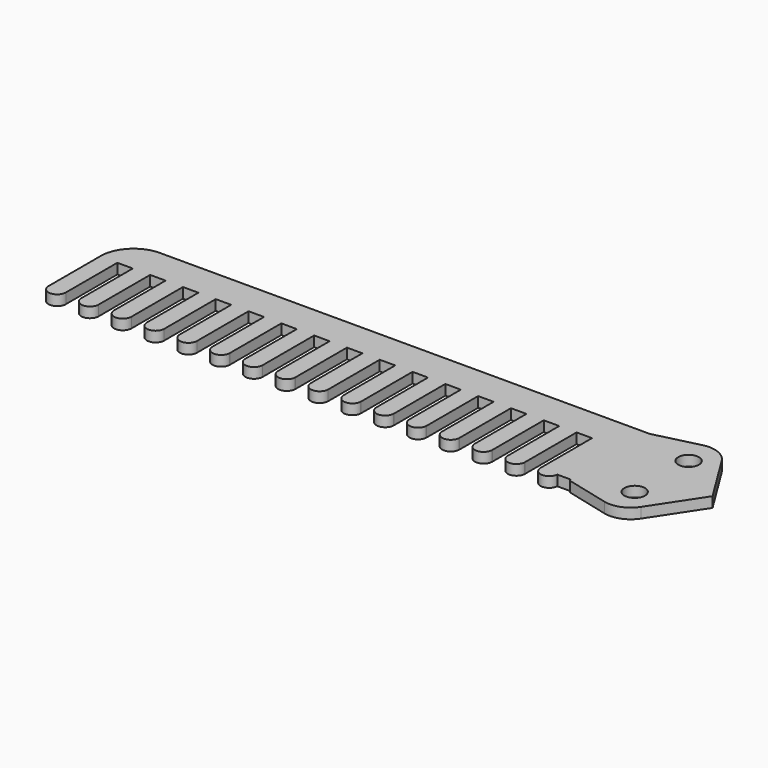
from build123d import *
from build123d import SkipClean  # not in build123d's __all__

# Parameters (mm, degrees)
F0_R     = 2
F1_DEPTH = 2
F3_DEPTH = 25.4
F4_DEPTH = 2
F5_DEPTH = 25.4


# Not quite as in the source:
# - a feature names something its author has since deleted; it is built from what else it names


with BuildPart() as f1:
    # F0 (on Top) → F1 (new body)
    with BuildSketch(Plane.XY):
        with BuildLine():
            ThreePointArc((-44.4982377637, 15.9537835574), (-46.6435438514, 15.0651686804), (-47.5321587284, 12.9198625927))
            Line((-47.5321587284, 12.9198625927), (-47.5321587284, 1.9581455603))
            ThreePointArc((-47.5321587284, 1.9581455603), (-46.0701489095, -1.5749303628), (-42.539108537, -3.0418496097))
            Line((-42.539108537, -3.0418496097), (58.6544047029, -3.182504855))
            ThreePointArc((58.6544047029, -3.182504855), (58.695576092, -3.383063352), (58.8128977225, -3.5508561677))
            Line((58.8128977225, -3.5508561677), (67.1425286707, -5.6492492557))
            ThreePointArc((67.1425286707, -5.6492492557), (70.1745553832, -5.4613941054), (72.5382215144, -3.553107449))
            Line((72.5382215144, -3.553107449), (78.7976136626, 5.9399087982))
            ThreePointArc((78.7976136626, 5.9399087982), (78.7234830832, 6.1327797263), (78.5951017421, 6.2946833056))
            Line((78.5951017421, 6.2946833056), (72.6648820615, 15.8458770867))
            ThreePointArc((72.6648820615, 15.8458770867), (70.3034587252, 17.8389512741), (67.2215312081, 18.0634232527))
            Line((67.2215312081, 18.0634232527), (58.6544042144, 15.9537835574))
            Line((58.6544042144, 15.9537835574), (-44.4982377637, 15.9537835574))
        make_face()
        with Locations((68.7303330245, -0.2896678891)):
            Circle(F0_R, mode=Mode.SUBTRACT)
        with Locations((68.7701961271, 12.7037232041)):
            Circle(F0_R, mode=Mode.SUBTRACT)
    extrude(amount=F1_DEPTH)

    # F2 (on face) → F3 (cut)
    with BuildSketch(Plane.XY.offset(2)):
        with BuildLine():
            Line((-10.789108537, 9.4149718061), (-13.784505137, 9.4149718061))
            Line((-13.784505137, 9.4149718061), (-13.784505137, -3.0465123845))
            ThreePointArc((-13.784505137, -3.0465123845), (-13.7845980378, -3.0641656349), (-13.7848767298, -3.0818169297))
            Line((-13.7848767298, -3.0818169297), (-10.7886505729, -3.0859815734))
            ThreePointArc((-10.7886505729, -3.0859815734), (-10.7890247148, -3.0639170979), (-10.789108537, -3.0418496097))
            Line((-10.789108537, -3.0418496097), (-10.789108537, 9.4149718061))
        make_face()
        with BuildLine():
            Line((-4.439108537, 9.4149718061), (-7.434505137, 9.4149718061))
            Line((-7.434505137, 9.4149718061), (-7.434505137, -3.0465123845))
            ThreePointArc((-7.434505137, -3.0465123845), (-7.4346503047, -3.0685795544), (-7.4350857828, -3.0906429046))
            Line((-7.4350857828, -3.0906429046), (-4.4384195675, -3.0948081599))
            ThreePointArc((-4.4384195675, -3.0948081599), (-4.4389730944, -3.0683316044), (-4.439108537, -3.0418496097))
            Line((-4.439108537, -3.0418496097), (-4.439108537, 9.4149718061))
        make_face()
        with BuildLine():
            Line((1.910891463, 9.4149718061), (-1.084505137, 9.4149718061))
            Line((-1.084505137, 9.4149718061), (-1.084505137, -3.0465123845))
            ThreePointArc((-1.084505137, -3.0465123845), (-1.0847141969, -3.0729939003), (-1.0853413245, -3.0994688148))
            Line((-1.0853413245, -3.0994688148), (1.911857947, -3.1036348111))
            ThreePointArc((1.911857947, -3.1036348111), (1.9110901561, -3.0727466615), (1.910891463, -3.0418496097))
            Line((1.910891463, -3.0418496097), (1.910891463, 9.4149718061))
        make_face()
        with BuildLine():
            Line((8.260891463, 9.4149718061), (5.265494863, 9.4149718061))
            Line((5.265494863, 9.4149718061), (5.265494863, -3.0465123845))
            ThreePointArc((5.265494863, -3.0465123845), (5.2652102793, -3.0774087645), (5.2643566248, -3.1082946604))
            Line((5.2643566248, -3.1082946604), (8.2622802241, -3.1124616635))
            ThreePointArc((8.2622802241, -3.1124616635), (8.2612141473, -3.0771629469), (8.260891463, -3.0418496097))
            Line((8.260891463, -3.0418496097), (8.260891463, 9.4149718061))
        make_face()
        with BuildLine():
            Line((14.610891463, 9.4149718061), (11.615494863, 9.4149718061))
            Line((11.615494863, 9.4149718061), (11.615494863, -3.0465123845))
            ThreePointArc((11.615494863, -3.0465123845), (11.6150740117, -3.0818246882), (11.6139098113, -3.1171203048))
            Line((11.6139098113, -3.1171203048), (14.6126631372, -3.1212884611))
            ThreePointArc((14.6126631372, -3.1212884611), (14.6113068287, -3.081579528), (14.610891463, -3.0418496097))
            Line((14.610891463, -3.0418496097), (14.610891463, 9.4149718061))
        make_face()
        with BuildLine():
            Line((17.9635023619, -3.1259460039), (20.9630926527, -3.1301153236))
            ThreePointArc((20.9630926527, -3.1301153236), (20.9614111694, -3.0859969529), (20.960891463, -3.0418496097))
            Line((20.960891463, -3.0418496097), (20.960891463, 9.4149718061))
            Line((20.960891463, 9.4149718061), (17.965494863, 9.4149718061))
            Line((17.965494863, 9.4149718061), (17.965494863, -3.0465123845))
            ThreePointArc((17.965494863, -3.0465123845), (17.9649690528, -3.0862409946), (17.9635023619, -3.1259460039))
        make_face()
        with BuildLine():
            Line((24.3130483101, -3.1347716382), (27.3135688072, -3.1389422508))
            ThreePointArc((27.3135688072, -3.1389422508), (27.3115271807, -3.0904153143), (27.310891463, -3.0418496097))
            Line((27.310891463, -3.0418496097), (27.310891463, 9.4149718061))
            Line((27.310891463, 9.4149718061), (24.315494863, 9.4149718061))
            Line((24.315494863, 9.4149718061), (24.315494863, -3.0465123845))
            ThreePointArc((24.315494863, -3.0465123845), (24.3148524325, -3.0906581124), (24.3130483101, -3.1347716382))
        make_face()
        with BuildLine():
            Line((30.6625476193, -3.1435972077), (33.6640916417, -3.147769243))
            ThreePointArc((33.6640916417, -3.147769243), (33.6616548753, -3.0948347051), (33.660891463, -3.0418496097))
            Line((33.660891463, -3.0418496097), (33.660891463, 9.4149718061))
            Line((33.660891463, 9.4149718061), (30.665494863, 9.4149718061))
            Line((30.665494863, 9.4149718061), (30.665494863, -3.0465123845))
            ThreePointArc((30.665494863, -3.0465123845), (30.6647241389, -3.0950761342), (30.6625476193, -3.1435972077))
        make_face()
        with BuildLine():
            Line((37.0120002484, -3.1524227123), (40.014661201, -3.1565963001))
            ThreePointArc((40.014661201, -3.1565963001), (40.011794267, -3.0992552184), (40.010891463, -3.0418496097))
            Line((40.010891463, -3.0418496097), (40.010891463, 9.4149718061))
            Line((40.010891463, 9.4149718061), (37.015494863, 9.4149718061))
            Line((37.015494863, 9.4149718061), (37.015494863, -3.0465123845))
            ThreePointArc((37.015494863, -3.0465123845), (37.0145841593, -3.0994951529), (37.0120002484, -3.1524227123))
        make_face()
        with BuildLine():
            Line((43.3614061528, -3.1612481519), (46.3652775338, -3.1654234222))
            ThreePointArc((46.3652775338, -3.1654234222), (46.361945371, -3.1036769476), (46.360891463, -3.0418496097))
            Line((46.360891463, -3.0418496097), (46.360891463, 9.4149718061))
            Line((46.360891463, 9.4149718061), (43.365494863, 9.4149718061))
            Line((43.365494863, 9.4149718061), (43.365494863, -3.0465123845))
            ThreePointArc((43.365494863, -3.0465123845), (43.3644324794, -3.1039152616), (43.3614061528, -3.1612481519))
        make_face()
        with BuildLine():
            Line((49.7107652838, -3.1700735266), (52.7159406928, -3.1742506094))
            ThreePointArc((52.7159406928, -3.1742506094), (52.7121082036, -3.1080999865), (52.710891463, -3.0418496097))
            Line((52.710891463, -3.0418496097), (52.710891463, 9.4149718061))
            Line((52.710891463, 9.4149718061), (49.715494863, 9.4149718061))
            Line((49.715494863, 9.4149718061), (49.715494863, -3.0465123845))
            ThreePointArc((49.715494863, -3.0465123845), (49.7142690839, -3.1083365537), (49.7107652838, -3.1700735266))
        make_face()
        with BuildLine():
            Line((-17.139108537, 9.4149718061), (-20.134505137, 9.4149718061))
            Line((-20.134505137, 9.4149718061), (-20.134505137, -3.0465123845))
            ThreePointArc((-20.134505137, -3.0465123845), (-20.1345573909, -3.0597520498), (-20.1347141494, -3.0729908903))
            Line((-20.1347141494, -3.0729908903), (-17.1388350895, -3.0771550515))
            ThreePointArc((-17.1388350895, -3.0771550515), (-17.1390647112, -3.0595030501), (-17.139108537, -3.0418496097))
            Line((-17.139108537, -3.0418496097), (-17.139108537, 9.4149718061))
        make_face()
        with BuildLine():
            Line((-23.489108537, 9.4149718061), (-26.484505137, 9.4149718061))
            Line((-26.484505137, 9.4149718061), (-26.484505137, -3.0465123845))
            ThreePointArc((-26.484505137, -3.0465123845), (-26.4845283601, -3.0553387076), (-26.4845980289, -3.0641647862))
            Line((-26.4845980289, -3.0641647862), (-23.4889731336, -3.0683285942))
            ThreePointArc((-23.4889731336, -3.0683285942), (-23.4890930885, -3.0550893691), (-23.489108537, -3.0418496097))
            Line((-23.489108537, -3.0418496097), (-23.489108537, 9.4149718061))
        make_face()
        with BuildLine():
            Line((-29.839108537, 9.4149718061), (-32.834505137, 9.4149718061))
            Line((-32.834505137, 9.4149718061), (-32.834505137, -3.0465123845))
            ThreePointArc((-32.834505137, -3.0465123845), (-32.8345109427, -3.0509255163), (-32.8345283597, -3.0553386176))
            Line((-32.8345283597, -3.0553386176), (-29.8390647178, -3.0595022015))
            ThreePointArc((-29.8390647178, -3.0595022015), (-29.8391098505, -3.0506759632), (-29.839108537, -3.0418496097))
            Line((-29.839108537, -3.0418496097), (-29.839108537, 9.4149718061))
        make_face()
        with BuildLine():
            Line((-36.189108537, 9.4149718061), (-39.184505137, 9.4149718061))
            Line((-39.184505137, 9.4149718061), (-39.184505137, -3.0465123845))
            Line((-39.184505137, -3.0465123845), (-36.1891098507, -3.0506758733))
            ThreePointArc((-36.1891098507, -3.0506758733), (-36.1891149995, -3.0462627406), (-36.189108537, -3.0418496097))
            Line((-36.189108537, -3.0418496097), (-36.189108537, 9.4149718061))
        make_face()
    extrude(amount=-F3_DEPTH, mode=Mode.SUBTRACT)

    # F2 (on face) → F4 (join)
    with BuildSketch(Plane.XY.offset(2)):
        with BuildLine():
            ThreePointArc((52.7159406928, -3.1742506094), (54.3858617756, -4.7214826971), (56.0600775884, -3.1788988362))
            Line((56.0600775884, -3.1788988362), (52.7159406928, -3.1742506094))
        make_face()
        with BuildLine():
            ThreePointArc((46.3652775338, -3.1654234222), (48.0358617756, -4.7214826971), (49.7107652838, -3.1700735266))
            Line((49.7107652838, -3.1700735266), (46.3652775338, -3.1654234222))
        make_face()
        with BuildLine():
            ThreePointArc((40.014661201, -3.1565963001), (41.6858617756, -4.7214826971), (43.3614061528, -3.1612481519))
            Line((43.3614061528, -3.1612481519), (40.014661201, -3.1565963001))
        make_face()
        with BuildLine():
            ThreePointArc((33.6640916417, -3.147769243), (35.3358617756, -4.7214826971), (37.0120002484, -3.1524227123))
            Line((37.0120002484, -3.1524227123), (33.6640916417, -3.147769243))
        make_face()
        with BuildLine():
            ThreePointArc((27.3135688072, -3.1389422508), (28.9858617756, -4.7214826971), (30.6625476193, -3.1435972077))
            Line((30.6625476193, -3.1435972077), (27.3135688072, -3.1389422508))
        make_face()
        with BuildLine():
            ThreePointArc((20.9630926527, -3.1301153236), (22.6358617756, -4.7214826971), (24.3130483101, -3.1347716382))
            Line((24.3130483101, -3.1347716382), (20.9630926527, -3.1301153236))
        make_face()
        with BuildLine():
            Line((17.9635023619, -3.1259460039), (14.6126631372, -3.1212884611))
            ThreePointArc((14.6126631372, -3.1212884611), (16.2858617756, -4.7214826971), (17.9635023619, -3.1259460039))
        make_face()
        with BuildLine():
            Line((11.6139098113, -3.1171203048), (8.2622802241, -3.1124616635))
            ThreePointArc((8.2622802241, -3.1124616635), (9.9358617756, -4.7214826971), (11.6139098113, -3.1171203048))
        make_face()
        with BuildLine():
            Line((5.2643566248, -3.1082946604), (1.911857947, -3.1036348111))
            ThreePointArc((1.911857947, -3.1036348111), (3.5858585328, -4.7238157048), (5.2643566248, -3.1082946604))
        make_face()
        with BuildLine():
            Line((-1.0853413245, -3.0994688148), (-4.4384195675, -3.0948081599))
            ThreePointArc((-4.4384195675, -3.0948081599), (-2.7641414672, -4.7238157048), (-1.0853413245, -3.0994688148))
        make_face()
        with BuildLine():
            Line((-7.4350857828, -3.0906429046), (-10.7886505729, -3.0859815734))
            ThreePointArc((-10.7886505729, -3.0859815734), (-9.1141414672, -4.7238157048), (-7.4350857828, -3.0906429046))
        make_face()
        with BuildLine():
            Line((-13.7848767298, -3.0818169297), (-17.1388350895, -3.0771550515))
            ThreePointArc((-17.1388350895, -3.0771550515), (-15.4641414672, -4.7238157048), (-13.7848767298, -3.0818169297))
        make_face()
        with BuildLine():
            Line((-20.1347141494, -3.0729908903), (-23.4889731336, -3.0683285942))
            ThreePointArc((-23.4889731336, -3.0683285942), (-21.8141414672, -4.7238157048), (-20.1347141494, -3.0729908903))
        make_face()
        with BuildLine():
            Line((-26.4845980289, -3.0641647862), (-29.8390647178, -3.0595022015))
            ThreePointArc((-29.8390647178, -3.0595022015), (-28.1641414672, -4.7238157048), (-26.4845980289, -3.0641647862))
        make_face()
        with BuildLine():
            Line((-32.8345283597, -3.0553386176), (-36.1891098507, -3.0506758733))
            ThreePointArc((-36.1891098507, -3.0506758733), (-34.5141414672, -4.7238157048), (-32.8345283597, -3.0553386176))
        make_face()
        with BuildLine():
            Line((-39.184505137, -3.0465123845), (-42.539108537, -3.0418496097))
            ThreePointArc((-42.539108537, -3.0418496097), (-40.8641414672, -4.7238157048), (-39.184505137, -3.0465123845))
        make_face()
    with SkipClean():  # cleaning this boolean's faces spoils the solid; the shape is the same uncleaned
        extrude(amount=-F4_DEPTH)

    # F2 (on face) → F5 (cut)
    with BuildSketch(Plane.XY.offset(2)):
        with BuildLine():
            ThreePointArc((-42.539108537, 9.6037835574), (-40.6792365975, 14.0939116179), (-36.189108537, 15.9537835574))
            Line((-36.189108537, 15.9537835574), (-44.4982377637, 15.9537835574))
            ThreePointArc((-44.4982377637, 15.9537835574), (-46.6435438514, 15.0651686804), (-47.5321587284, 12.9198625927))
            Line((-47.5321587284, 12.9198625927), (-47.5321587284, 1.9581455603))
            ThreePointArc((-47.5321587284, 1.9581455603), (-46.0701489095, -1.5749303628), (-42.539108537, -3.0418496097))
            Line((-42.539108537, -3.0418496097), (-42.539108537, 9.4149718061))
            Line((-42.539108537, 9.4149718061), (-42.539108537, 9.6037835574))
        make_face()
    extrude(amount=-F5_DEPTH, mode=Mode.SUBTRACT)


solid = f1.part
